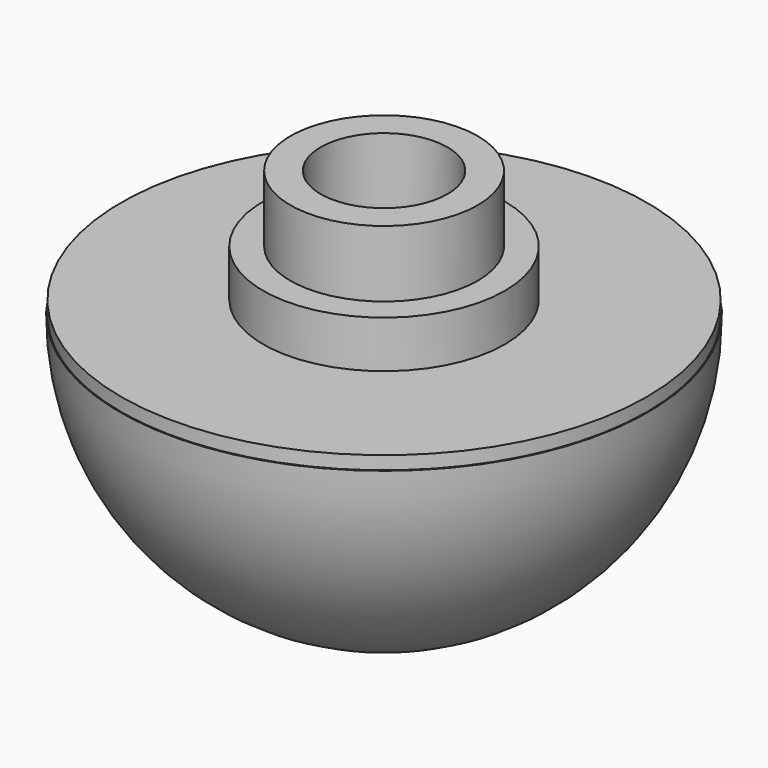
from build123d import *

# Parameters (mm, degrees)
F0_R     = 3.937
F0_R_2   = 2.667
F1_DEPTH = 2.794
F2_R     = 5.08
F3_DEPTH = 1.9812
F4_R     = 11.049
F5_DEPTH = 1.524


# Not quite as in the source:
# - a feature names something its author has since deleted; it is built from what else it names


with BuildPart() as f1:
    # F0 (on Top) → F1 (new body)
    with BuildSketch(Plane.XY):
        Circle(F0_R)
        Circle(F0_R_2, mode=Mode.SUBTRACT)
    extrude(amount=F1_DEPTH)

    # F2 (on face) → F3 (join)
    with BuildSketch(Plane(origin=(0, 0, 0), x_dir=(1, 0, 0), z_dir=(0, 0, -1))):
        Circle(F2_R)
    extrude(amount=F3_DEPTH)

    # F4 (on face) → F5 (join)
    with BuildSketch(Plane(origin=(0, 0, -1.9812), x_dir=(1, 0, 0), z_dir=(0, 0, -1))):
        Circle(F4_R)
    extrude(amount=F5_DEPTH)

    # F6 (on Front) → F7 (revolve)
    with BuildSketch(Plane.XZ):
        with BuildLine():
            Line((0, -2.54), (-11.09184091, -2.54))
            ThreePointArc((-11.09184091, -2.54), (-7.8431159233, -10.3831159233), (0, -13.63184091))
            Line((0, -13.63184091), (0, -3.5557490773))
            Line((0, -3.5557490773), (0, -2.54))
        make_face()
    revolve(axis=Axis((0, 0, -8.5937949937), (0, 0, -1)))


solid = f1.part
